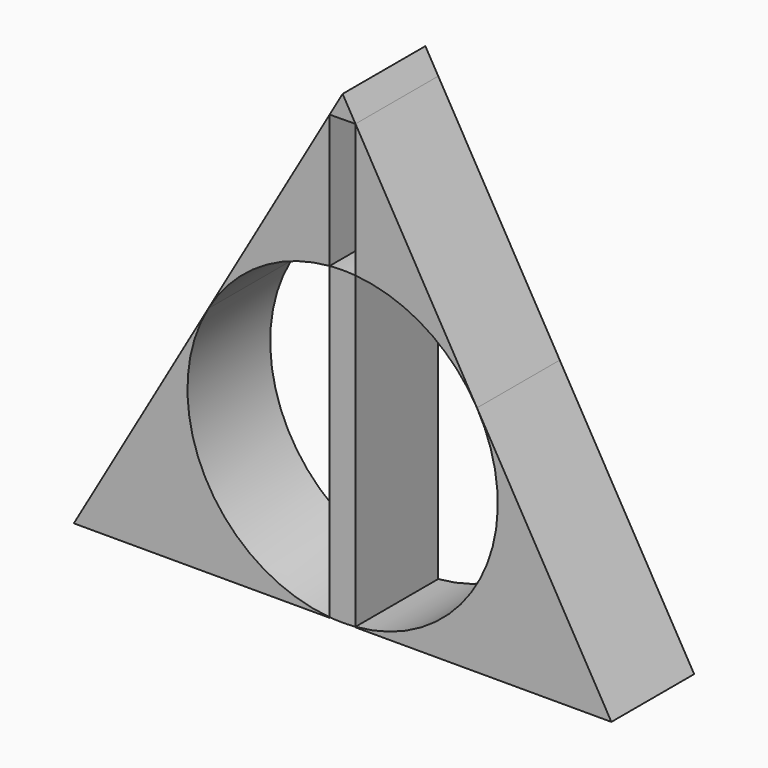
from build123d import *

# Parameters (mm, degrees)
F1_DEPTH = 25.4


with BuildPart() as f1:
    # F0 (on Front) → F1 (new body)
    with BuildSketch(Plane.XZ):
        Polygon((-3.1914482743, 70.6722494391), (3.1582920346, 70.7296777309), (0, 76.2), align=None)
    extrude(amount=F1_DEPTH)


with BuildPart() as f1b:
    # F0 (on Front) → F1, piece 2 (new body)
    with BuildSketch(Plane.XZ):
        with BuildLine():
            ThreePointArc((-32.9955673517, 19.0500009224), (-20.4164079771, 32.168000953), (-3.1914482743, 37.9660987976))
            Line((-3.1914482743, 37.9660987976), (-3.1914482743, 70.6722494391))
            Line((-3.1914482743, 70.6722494391), (-32.9955673517, 19.0500009224))
        make_face()
    extrude(amount=F1_DEPTH)


with BuildPart() as f1c:
    # F0 (on Front) → F1, piece 3 (new body)
    with BuildSketch(Plane.XZ):
        with BuildLine():
            ThreePointArc((3.1582920346, 37.9688713478), (20.4023610122, 32.1769119887), (32.995568315, 19.0499992538))
            Line((32.995568315, 19.0499992538), (3.1582920346, 70.7296777309))
            Line((3.1582920346, 70.7296777309), (3.1582920346, 37.9688713478))
        make_face()
    extrude(amount=F1_DEPTH)


with BuildPart() as f1d:
    # F0 (on Front) → F1, piece 4 (new body)
    with BuildSketch(Plane.XZ):
        with BuildLine():
            ThreePointArc((4.21e-08, -38.1), (1.58050653, -38.0672037206), (3.1582920346, -37.9688713478))
            Line((3.1582920346, -37.9688713478), (3.1582920346, 37.9688713478))
            ThreePointArc((3.1582920346, 37.9688713478), (-0.0166359796, 38.099996368), (-3.1914482743, 37.9660987976))
            Line((-3.1914482743, 37.9660987976), (-3.1914482743, -37.9660987976))
            ThreePointArc((-3.1914482743, -37.9660987976), (-1.5971279966, -38.0665099814), (4.21e-08, -38.1))
        make_face()
    extrude(amount=F1_DEPTH)


with BuildPart() as f1e:
    # F0 (on Front) → F1, piece 5 (new body)
    with BuildSketch(Plane.XZ):
        with BuildLine():
            Line((-3.1914482743, -38.1), (-3.1914482743, -37.9660987976))
            ThreePointArc((-3.1914482743, -37.9660987976), (-33.7651289321, -17.6501010819), (-32.9955673517, 19.0500009224))
            Line((-32.9955673517, 19.0500009224), (-65.9911357684, -38.1))
            Line((-65.9911357684, -38.1), (-3.1914482743, -38.1))
        make_face()
    extrude(amount=F1_DEPTH)


with BuildPart() as f1f:
    # F0 (on Front) → F1, piece 6 (new body)
    with BuildSketch(Plane.XZ):
        with BuildLine():
            ThreePointArc((32.995568315, 19.0499992538), (36.8017740931, 9.8610052023), (38.1, 0))
            ThreePointArc((38.1, 0), (28.0351647625, -25.7999910221), (3.1582920346, -37.9688713478))
            Line((3.1582920346, -37.9688713478), (3.1582920346, -38.1))
            Line((3.1582920346, -38.1), (65.9911357684, -38.1))
            Line((65.9911357684, -38.1), (32.995568315, 19.0499992538))
        make_face()
    extrude(amount=F1_DEPTH)


solid = Compound([f1.part, f1b.part, f1c.part, f1d.part, f1e.part, f1f.part])
